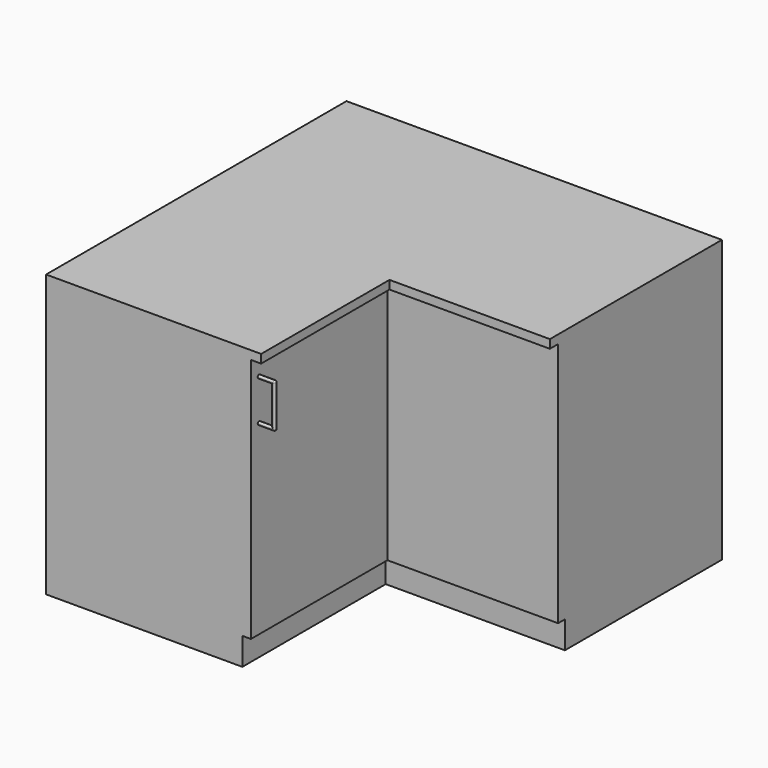
from build123d import *

# Parameters (mm, degrees)
F0_W        = 600
F0_H        = 500
F1_DEPTH    = 800
F2_W        = 500
F2_H        = 80
F3_DEPTH    = 25
F5_DEPTH    = 50
F6_T1_DEPTH = 145.0048285071
F6_T4_ANGLE = 180
F6_T6_ANGLE = 180
F7_W        = 40
F7_H        = 110
F8_DEPTH    = 25
F9_R        = 4.99999
F10_W       = 630
F10_H       = 500
F11_DEPTH   = 25
F12_DEPTH   = 600
F13_W       = 600
F13_H       = 800
F14_DEPTH   = 500
F15_W       = 630
F15_H       = 25
F16_DEPTH   = 470
F17_W       = 500
F17_H       = 80
F18_DEPTH   = 25
F19_W       = 575
F19_H       = 80
F20_DEPTH   = 25


# Not quite as in the source:
# - a fillet or chamfer that OpenCascade refuses, or shapes differently, is made with other operations: its cross-section is extruded or revolved along the edge and cut away or added
# - a fillet or chamfer is up to 0.001 mm smaller than in the source, because OpenCascade refuses the exact size


with BuildPart() as f1:
    # F0 (on Top) → F1 (new body)
    with BuildSketch(Plane.XY):
        Rectangle(F0_W, F0_H)
    extrude(amount=F1_DEPTH)

    # F2 (on face) → F3 (cut)
    with BuildSketch(Plane.YZ.offset(300)):
        with Locations((0, 40)):
            Rectangle(F2_W, F2_H)
    extrude(amount=-F3_DEPTH, mode=Mode.SUBTRACT)

    # F4 (on face) → F5 (join)
    with BuildSketch(Plane.YZ.offset(300)):
        with BuildLine():
            ThreePointArc((-220, 750), (-223.5355339059, 748.5355339059), (-225, 745))
            Line((-225, 745), (-225, 625))
            ThreePointArc((-225, 625), (-223.5355339059, 621.4644660941), (-220, 620))
            ThreePointArc((-220, 620), (-216.4644660941, 621.4644660941), (-215, 625))
            Line((-215, 625), (-215, 745))
            ThreePointArc((-215, 745), (-216.4644660941, 748.5355339059), (-220, 750))
        make_face()
    extrude(amount=F5_DEPTH)

    # F6: fillet of radius 5 on 4 edges, made by hand

    # F6_s2 → F6_t1 (cut)
    with BuildSketch(Plane.XY.offset(612.4975857464)):
        with BuildLine():
            ThreePointArc((344.9990343146, -225.0004), (348.5355339059, -223.5355339059), (350.0004, -219.9990343146))
            Line((350.0004, -219.9990343146), (350.5005365685, -219.9990343146))
            ThreePointArc((350.5005365685, -219.9990343146), (350.5001365685, -222.4995171573), (350.5001365685, -225))
            Line((350.5001365685, -225), (350, -225.5001365685))
            ThreePointArc((350, -225.5001365685), (347.4995171573, -225.5001365685), (344.9990343146, -225.5005365685))
            Line((344.9990343146, -225.5005365685), (344.9990343146, -225.0004))
        make_face()
        with BuildLine():
            ThreePointArc((344.9990343146, -214.9996), (348.5355339059, -216.4644660941), (350.0004, -220.0009656854))
            Line((350.0004, -220.0009656854), (350.5005365685, -220.0009656854))
            ThreePointArc((350.5005365685, -220.0009656854), (350.5001365685, -217.5004828427), (350.5001365685, -215))
            Line((350.5001365685, -215), (350, -214.4998634315))
            ThreePointArc((350, -214.4998634315), (347.4995171573, -214.4998634315), (344.9990343146, -214.4994634315))
            Line((344.9990343146, -214.4994634315), (344.9990343146, -214.9996))
        make_face()
    extrude(amount=F6_T1_DEPTH, mode=Mode.SUBTRACT)

    # F6_s3 → F6_t4 (revolve, cut)
    with BuildSketch(Plane.XY.offset(745)):
        with BuildLine():
            ThreePointArc((344.9990343146, -225.0004), (348.5351924681, -223.5358753108), (350.0003999068, -220))
            Line((350.0003999068, -220), (350.5005364913, -220))
            Line((350.5005364913, -220), (350.5001365685, -225))
            Line((350.5001365685, -225), (350, -225.5001365685))
            ThreePointArc((350, -225.5001365685), (347.4995171573, -225.5001365685), (344.9990343146, -225.5005365685))
            Line((344.9990343146, -225.5005365685), (344.9990343146, -225.0004))
        make_face()
    revolve(axis=Axis((350, -220, 745), (-1, 0, 0)), revolution_arc=F6_T4_ANGLE, mode=Mode.SUBTRACT)

    # F6_s5 → F6_t6 (revolve, cut)
    with BuildSketch(Plane.XY.offset(625)):
        with BuildLine():
            ThreePointArc((344.9990343146, -214.9996), (348.5351924681, -216.4641246892), (350.0003999068, -220))
            Line((350.0003999068, -220), (350.5005364913, -220))
            Line((350.5005364913, -220), (350.5001365685, -215))
            Line((350.5001365685, -215), (350, -214.4998634315))
            ThreePointArc((350, -214.4998634315), (347.4995171573, -214.4998634315), (344.9990343146, -214.4994634315))
            Line((344.9990343146, -214.4994634315), (344.9990343146, -214.9996))
        make_face()
    revolve(axis=Axis((350, -220, 625), (-1, 0, 0)), revolution_arc=F6_T6_ANGLE, mode=Mode.SUBTRACT)

    # F7 (on face) → F8 (cut)
    with BuildSketch(Plane(origin=(0, -215, 0), x_dir=(-1, 0, 0), z_dir=(0, 1, 0))):
        with Locations((-320, 685)):
            Rectangle(F7_W, F7_H)
    extrude(amount=-F8_DEPTH, mode=Mode.SUBTRACT)

    # F9 (radius 5 in the source; OpenCascade refuses exactly that, so slightly less here)
    f9_edges = [f1.edges().sort_by_distance(p)[0] for p in [
        (320, -215, 740),
        (340, -215, 685),
        (320, -215, 630),
        (320, -225, 740),
        (340, -225, 685),
        (320, -225, 630),
    ]]
    fillet(f9_edges, radius=F9_R)

    # F10 (on face) → F11 (join)
    with BuildSketch(Plane.XY.offset(800)):
        with Locations((15, 0)):
            Rectangle(F10_W, F10_H)
    extrude(amount=F11_DEPTH)

    # F12 (add): a face of the model
    f12_faces = [f1.faces().sort_by_distance(p)[0] for p in [
        (-0.6860759494, 250, 414.6164556962),
    ]]
    extrude(f12_faces, amount=F12_DEPTH)

    # F13 (on face) → F14 (join)
    with BuildSketch(Plane.YZ.offset(300)):
        with Locations((550, 400)):
            Rectangle(F13_W, F13_H)
    extrude(amount=F14_DEPTH)

    # F15 (on face) → F16 (join)
    with BuildSketch(Plane.YZ.offset(330)):
        with Locations((535, 812.5)):
            Rectangle(F15_W, F15_H)
    extrude(amount=F16_DEPTH)

    # F17 (on face) → F18 (cut)
    with BuildSketch(Plane.XZ.offset(-250)):
        with Locations((550, 40)):
            Rectangle(F17_W, F17_H)
    extrude(amount=-F18_DEPTH, mode=Mode.SUBTRACT)

    # F19 (on face) → F20 (join)
    with BuildSketch(Plane(origin=(300, 0, 0), x_dir=(0, -1, 0), z_dir=(-1, 0, 0))):
        with Locations((-562.5, 40)):
            Rectangle(F19_W, F19_H)
    extrude(amount=F20_DEPTH)


solid = f1.part
